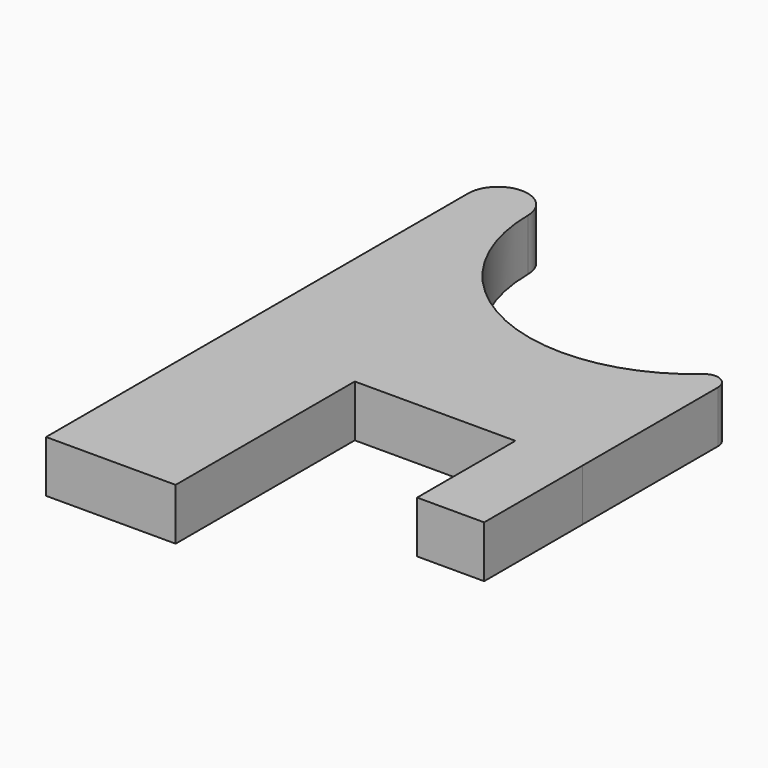
from build123d import *

# Parameters (mm, degrees)
F1_DEPTH = 5
F2_W     = 6.4714387385
F2_H     = 11.8567999452
F2_W_2   = 12.5
F2_H_2   = 9.7434073687
F3_DEPTH = 5


# Not quite as in the source:
# - ends of sketch curves that miss each other by under 0.0002 mm in the source are joined
# - a feature names something its author has since deleted; it is built from what else it names


with BuildPart() as f1:
    # F0 (on Top) → F1 (new body)
    with BuildSketch(Plane.XY):
        with BuildLine():
            Line((0, 29.2999204248), (0, 0))
            Line((0, 0), (34.4714387385, 0))
            Line((34.4714387385, 0), (34.4714387385, 16.3473710418))
            ThreePointArc((34.4714387385, 16.3473710418), (32.5790927131, 15.1300794804), (32.2559916738, 17.3568210333))
            ThreePointArc((32.2559916738, 17.3568210333), (15.182844974, 14.8438668457), (5.7578901922, 29.2999210911))
            ThreePointArc((5.7578901922, 29.2999210911), (2.8789043427, 26.4210160822), (0, 29.2999204248))
        make_face()
        with BuildLine():
            ThreePointArc((5.7577396052, 29.3198639813), (2.8689325046, 32.1788074974), (0, 29.2999204248))
            ThreePointArc((0, 29.2999204248), (2.8789043427, 26.4210160822), (5.7578086853, 29.2999204248))
            ThreePointArc((5.7578086853, 29.2999204248), (5.7578117914, 29.3098925127), (5.7577396052, 29.3198639813))
        make_face()
        with BuildLine():
            ThreePointArc((32.2559916738, 17.3568210333), (32.5790927131, 15.1300794804), (34.4714387385, 16.3473710418))
            ThreePointArc((34.4714387385, 16.3473710418), (33.6883902233, 17.5646626032), (32.2559916738, 17.3568210333))
        make_face()
    extrude(amount=F1_DEPTH)

    # F2 (on face) → F3 (join)
    with BuildSketch(Plane.XY.offset(5)):
        with BuildLine():
            Line((28, 0), (34.4714387385, 0))
            Line((34.4714387385, 0), (34.4714387385, 16.3473710418))
            ThreePointArc((34.4714387385, 16.3473710418), (33.6883902233, 17.5646626032), (32.2559916738, 17.3568210333))
            ThreePointArc((32.2559916738, 17.3568210333), (15.182844974, 14.8438668457), (5.7578901922, 29.2999210911))
            ThreePointArc((5.7578901922, 29.2999210911), (5.757811792, 29.3098923335), (5.7577396052, 29.3198639813))
            ThreePointArc((5.7577396052, 29.3198639813), (2.8689325046, 32.1788074974), (0, 29.2999204248))
            Line((0, 29.2999204248), (0, 25.3991372883))
            Line((0, 25.3991372883), (0, 0))
            Line((0, 0), (12.5, 0))
            Line((12.5, 0), (28, 0))
        make_face()
        with Locations((31.2357193692, -5.9283999726)):
            Rectangle(F2_W, F2_H)
        with Locations((6.25, -5.9283999726)):
            Rectangle(F2_W_2, F2_H)
        with Locations((6.25, -16.7285036296)):
            Rectangle(F2_W_2, F2_H_2)
        with Locations((6.25, -5.9283999726)):
            Rectangle(F2_W_2, F2_H)
    extrude(amount=-F3_DEPTH)


solid = f1.part
